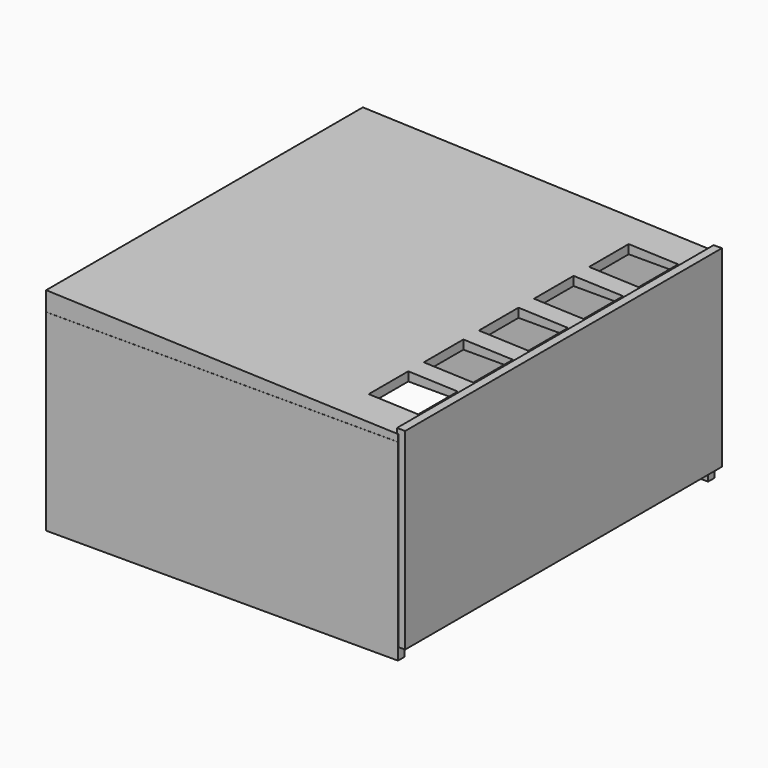
from build123d import *

# Parameters (mm, degrees)
F0_W        = 18
F0_H        = 18
F3_DEPTH    = 7
F4_T1_DEPTH = 809.5850048039
F5_START    = 42
F1_W        = 128
F1_H        = 70
F5_DEPTH    = 3
F6_START    = -96
F6_DEPTH    = 3
F7_START    = 55
F2_W        = 144
F2_H        = 70
F7_DEPTH    = 3


# Not quite as in the source:
# - a fillet or chamfer that OpenCascade refuses, or shapes differently, is made with other operations: its cross-section is extruded or revolved along the edge and cut away or added


with BuildPart() as f3:
    # F0 (on Top) → F3 (new body)
    with BuildSketch(Plane.XY):
        Polygon((52.5088317096, 99.0367529392), (-72.4911682904, 99.0367529392), (-72.4911682904, -44.9632470608), (52.5088317096, -44.9632470608), (55.5088317096, -44.9632470608), (55.5088317096, 99.0367529392), align=None)
        with Locations((43.5088317096, -23.0649668574)):
            Rectangle(F0_W, F0_H, mode=Mode.SUBTRACT)
        with Locations((43.5088317096, 1.9858930409)):
            Rectangle(F0_W, F0_H, mode=Mode.SUBTRACT)
        with Locations((43.5088317096, 27.0367529392)):
            Rectangle(F0_W, F0_H, mode=Mode.SUBTRACT)
        with Locations((43.5088317096, 52.0876128376)):
            Rectangle(F0_W, F0_H, mode=Mode.SUBTRACT)
        with Locations((43.5088317096, 77.1384727359)):
            Rectangle(F0_W, F0_H, mode=Mode.SUBTRACT)
    extrude(amount=F3_DEPTH)

    # F4: chamfer of 128 x 4.4698584949 on 1 edges, made by hand

    # F4_s2 → F4_t1 (cut)
    with BuildSketch(Plane.XZ.offset(-431.8292553412)):
        Polygon((-72.4911682904, 7), (55.5088317096, 2.5301415051), (55.5088317096, 7), align=None)
    extrude(amount=F4_T1_DEPTH, mode=Mode.SUBTRACT)

    # F1 (on Front) → F6 (join)
    with BuildSketch(Plane.XZ.offset(F6_START)):
        with Locations((-8.4911682904, -35)):
            Rectangle(F1_W, F1_H)
    extrude(amount=-F6_DEPTH)


with BuildPart() as f5:
    # F1 (on Front) → F5 (new body)
    with BuildSketch(Plane.XZ.offset(F5_START)):
        with Locations((-8.4911682904, -35)):
            Rectangle(F1_W, F1_H)
    extrude(amount=F5_DEPTH)


with BuildPart() as f7:
    # F2 (on Right) → F7 (new body)
    with BuildSketch(Plane.YZ.offset(F7_START)):
        with Locations((27.1626058966, -30.7089579414)):
            Rectangle(F2_W, F2_H)
    extrude(amount=F7_DEPTH)


solid = Compound([f3.part, f5.part, f7.part])
